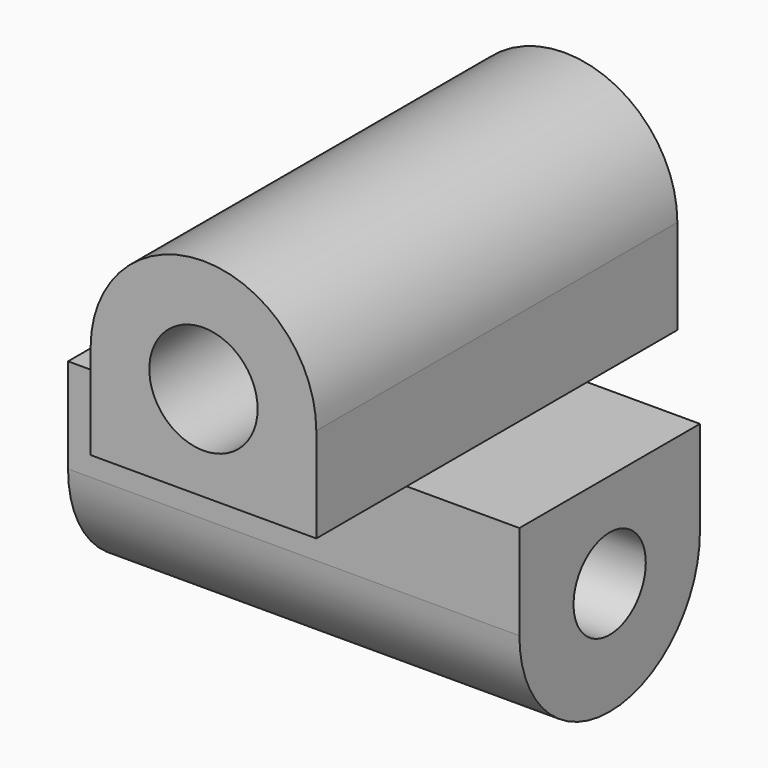
from build123d import *

# Parameters (mm, degrees)
F0_R     = 6
F1_DEPTH = 25
F2_R     = 5
F3_DEPTH = 25


# Not quite as in the source:
# - a feature names something its author has since deleted; it is built from what else it names


with BuildPart() as f1:
    # F0 (on Front) → F1 (new body, symmetric)
    with BuildSketch(Plane.XZ):
        with BuildLine():
            ThreePointArc((6.7823299831, 9.5), (10.9779124789, 14.0220875211), (12.5, 20))
            ThreePointArc((12.5, 20), (0, 32.5), (-12.5, 20))
            ThreePointArc((-12.5, 20), (-10.9779124789, 14.0220875211), (-6.7823299831, 9.5))
            Line((-6.7823299831, 9.5), (6.7823299831, 9.5))
        make_face()
        with Locations((0, 20)):
            Circle(F0_R, mode=Mode.SUBTRACT)
        with BuildLine():
            Line((12.5, 9.5), (12.5, 20))
            ThreePointArc((12.5, 20), (10.9779124789, 14.0220875211), (6.7823299831, 9.5))
            Line((6.7823299831, 9.5), (12.5, 9.5))
        make_face()
        with BuildLine():
            ThreePointArc((-6.7823299831, 9.5), (-10.9779124789, 14.0220875211), (-12.5, 20))
            Line((-12.5, 20), (-12.5, 9.5))
            Line((-12.5, 9.5), (-6.7823299831, 9.5))
        make_face()
    extrude(amount=F1_DEPTH, both=True)

    # F2 (on Right) → F3 (join, symmetric)
    with BuildSketch(Plane.YZ):
        with BuildLine():
            ThreePointArc((-6.7823299831, 9.5), (-10.9779124789, 4.9779124789), (-12.5, -1))
            ThreePointArc((-12.5, -1), (0, -13.5), (12.5, -1))
            ThreePointArc((12.5, -1), (10.9779124789, 4.9779124789), (6.7823299831, 9.5))
            Line((6.7823299831, 9.5), (-6.7823299831, 9.5))
        make_face()
        with Locations((0, -1)):
            Circle(F2_R, mode=Mode.SUBTRACT)
        with BuildLine():
            Line((-12.5, 9.5), (-12.5, -1))
            ThreePointArc((-12.5, -1), (-10.9779124789, 4.9779124789), (-6.7823299831, 9.5))
            Line((-6.7823299831, 9.5), (-12.5, 9.5))
        make_face()
        with BuildLine():
            ThreePointArc((6.7823299831, 9.5), (10.9779124789, 4.9779124789), (12.5, -1))
            Line((12.5, -1), (12.5, 9.5))
            Line((12.5, 9.5), (6.7823299831, 9.5))
        make_face()
    extrude(amount=F3_DEPTH, both=True)


solid = f1.part
